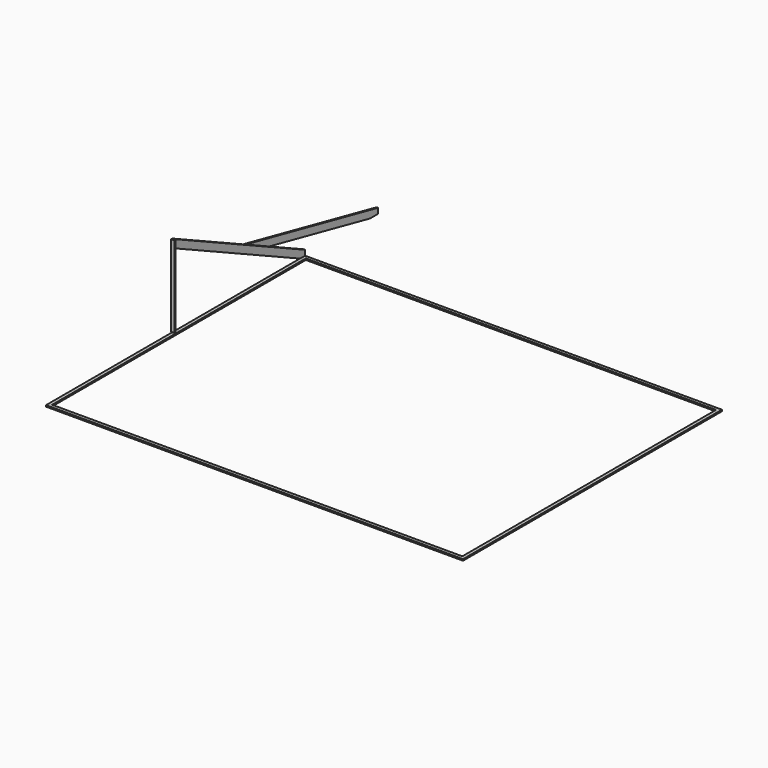
from build123d import *

# Parameters (mm, degrees)
F0_W     = 88.9
F0_H     = 8305.8
F1_DEPTH = 38.1
F3_DEPTH = 38.1
F6_DEPTH = 38.1
F2_W     = 19.05
F2_H     = 1422.4
F7_DEPTH = 88.9


with BuildPart() as f1:
    # F0 (on Top) → F1 (new body)
    with BuildSketch(Plane.XY):
        Polygon((34.2559893398, 0), (34.2559893398, -82.0349754334), (123.1559893398, -82.0349754333), (2774.9563753398, -82.0349754333), (2863.8563753398, -82.0349754333), (10867.3559893398, -82.0349754333), (10956.2559893398, -82.0349754333), (10956.2559893398, 0), align=None)
        with Locations((78.7059893398, -4234.9349754334)):
            Rectangle(F0_W, F0_H)
        Polygon((123.1559893398, -8387.8349754334), (34.2559893398, -8387.8349754334), (34.2559893398, -8476.7349754334), (10956.2559893398, -8476.7349754334), (10956.2559893398, -8387.8349754334), (10867.3559893398, -8387.8349754334), (2829.600386, -8387.8349754334), (2740.700386, -8387.8349754333), align=None)
        with Locations((10911.8059893398, -4234.9349754334)):
            Rectangle(F0_W, F0_H)
    extrude(amount=F1_DEPTH)

    # F2 (on Right) → F3 (join)
    with BuildSketch(Plane.YZ):
        Polygon((-4304.7849754334, 2170.231597737), (-4304.7849754334, 1961.6500800771), (-4293.965460335, 1955.0110555127), (-4290.8496340128, 1953.0991354956), (-82.0349754333, 0), (-82.0349754334, 1.9344240427), (-82.0349754334, 38.1), (0, 38.1), (0, 162.5593582531), (0, 173.9197075367), (-7.2166001264, 177.4147298146), (-4304.7849754334, 2171.7), (-4304.7849754334, 2170.9657988685), align=None)
    extrude(amount=F3_DEPTH)

    # F5 (on face) → F6 (join)
    with BuildSketch(Plane.YZ):
        Polygon((2175.9779277023, 0), (2438.4, 0), (2438.4, 139.7), (-1899.566832523, 1055.559267592), (-1128.1700381134, 697.5928246615), align=None)
        Polygon((-1128.1700381134, 697.5928246615), (-1899.566832523, 1055.559267592), (-1902.4696932972, 1056.1721381014), (-1131.0728988876, 698.2056951709), align=None)
        Polygon((-1131.0728988876, 698.2056951709), (-1902.4696932972, 1056.1721381014), (-1905.3725540714, 1056.7850086108), (-1133.9757596618, 698.8185656803), align=None)
        Polygon((-1133.9757596618, 698.8185656803), (-1905.3725540714, 1056.7850086108), (-2730.6478288415, 1231.0223962843), (-1959.2510344318, 873.0559533537), align=None)
        Polygon((-1959.2510344318, 873.0559533537), (-2730.6478288415, 1231.0223962843), (-2733.5506896157, 1231.6352667937), (-1962.153895206, 873.6688238632), align=None)
        Polygon((-1962.153895206, 873.6688238632), (-2733.5506896157, 1231.6352667937), (-2736.4535503898, 1232.2481373031), (-1965.0567559802, 874.2816943726), align=None)
        Polygon((-1965.0567559802, 874.2816943726), (-2736.4535503898, 1232.2481373031), (-2738.2960922849, 1232.6371465177), (-1966.8992978753, 874.6707035872), align=None)
    extrude(amount=-F6_DEPTH)

    # F2 (on Right) → F7 (join)
    with BuildSketch(Plane.YZ):
        Polygon((-4323.8349754334, 1460.5), (-4304.7849754334, 1460.5), (-4304.7849754334, 1961.6500800771), (-4304.7849754334, 2170.231597737), (-4307.9492966175, 2171.7), (-4323.8349754334, 2171.7), align=None)
        Polygon((-4342.8849754334, 1460.5), (-4323.8349754334, 1460.5), (-4323.8349754334, 2171.7), (-4339.7206542492, 2171.7), (-4342.8849754334, 2170.231597737), (-4342.8849754334, 1961.6500800771), align=None)
        with Locations((-4314.3099754334, 749.3)):
            Rectangle(F2_W, F2_H)
        with Locations((-4333.3599754334, 749.3)):
            Rectangle(F2_W, F2_H)
    extrude(amount=F7_DEPTH)


solid = f1.part
